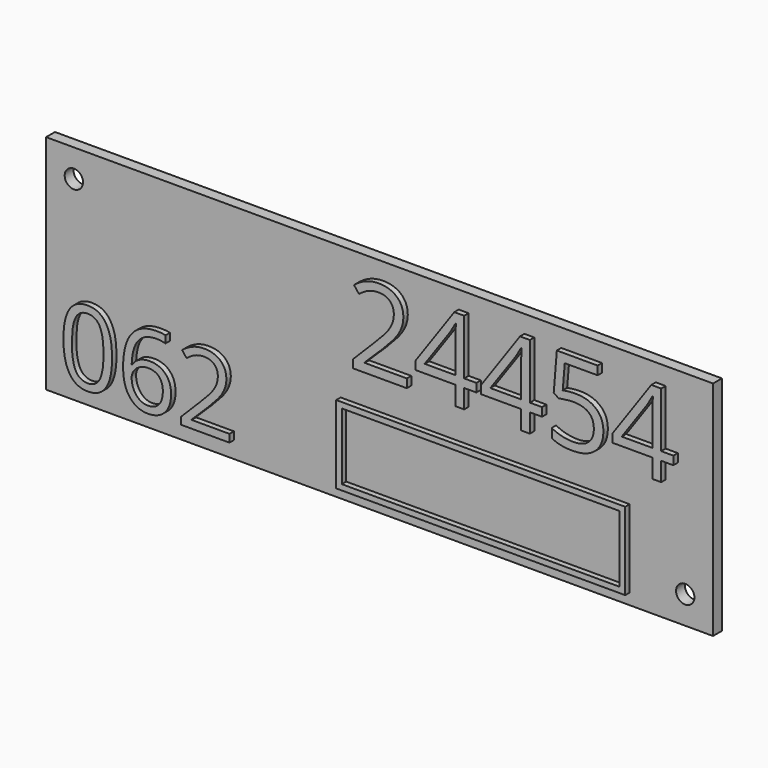
from build123d import *

# Parameters (mm, degrees)
F0_W         = 120
F0_H         = 40
F1_DEPTH     = 2
F3_D         = 3.3
F4_TEXT_SIZE = 20.6651598321
F5_DEPTH     = 1
F6_TEXT_SIZE = 18.5356140827
F7_DEPTH     = 1
F8_W         = 52
F8_H         = 14
F8_W_2       = 49.99999962
F8_H_2       = 11.99999962
F9_DEPTH     = 1


# Not quite as in the source:
# - Text() gives the source's letters only with a copy of the font that has no kerning and outlines rounded to 1/6400 em; it was checked with that copy


with BuildPart() as f1:
    # F0 (on Front) → F1 (new body)
    with BuildSketch(Plane.XZ):
        Rectangle(F0_W, F0_H)
    extrude(amount=F1_DEPTH)

    # F3 (through all)
    with Locations(Plane.XZ.offset(2)):
        with Locations((-55, 15), (55, -15)):
            Hole(F3_D / 2)

    # F4 (on face) → F5 (join)
    with BuildSketch(Plane.XZ.offset(2)):
        with Locations((-5, 2)):
            Text('24454', F4_TEXT_SIZE, font='Open Sans', text_align=(TextAlign.LEFT, TextAlign.BOTTOM))
    extrude(amount=F5_DEPTH)

    # F6 (on face) → F7 (join)
    with BuildSketch(Plane.XZ.offset(2)):
        with Locations((-57, -17)):
            Text('062', F6_TEXT_SIZE, font='Open Sans', text_align=(TextAlign.LEFT, TextAlign.BOTTOM))
    extrude(amount=F7_DEPTH)

    # F8 (on face) → F9 (join)
    with BuildSketch(Plane.XZ.offset(2)):
        with Locations((19, -11)):
            Rectangle(F8_W, F8_H)
        with Locations((19, -11)):
            Rectangle(F8_W_2, F8_H_2, mode=Mode.SUBTRACT)
    extrude(amount=F9_DEPTH)


solid = f1.part
